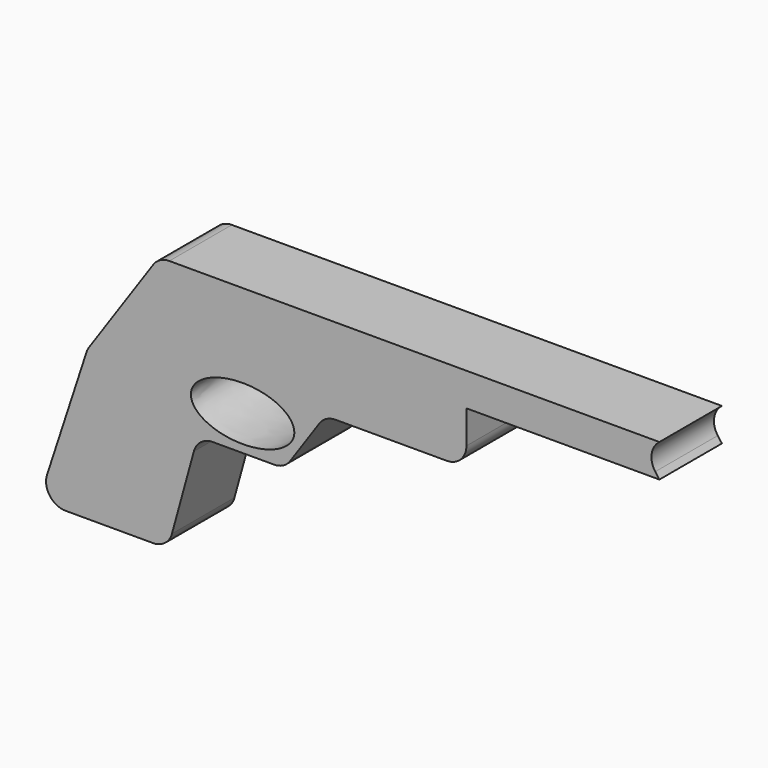
from build123d import *

# Parameters (mm, degrees)
F1_DEPTH = 25.4
F3_DEPTH = 25.4
F4_DEPTH = 25.4


# Not quite as in the source:
# - a feature names something its author has since deleted; it is built from what else it names


with BuildPart() as f1:
    # F0 (on Front) → F1 (new body)
    with BuildSketch(Plane.XZ):
        with BuildLine():
            Line((84.3741819263, 30.5474363267), (21.6592755169, 30.5474363267))
            Line((21.6592755169, 30.5474363267), (21.6592755169, 19.7983730762))
            Line((21.6592755169, 19.7983730762), (84.3741819263, 19.7983730762))
            Line((84.3741819263, 19.7983730762), (83.0258661007, 21.6186676974))
            ThreePointArc((83.0258661007, 21.6186676974), (81.8166137912, 26.0927593628), (83.9697137101, 30.196897289))
            Line((83.9697137101, 30.196897289), (84.3741819263, 30.5474363267))
        make_face()
        with BuildLine():
            Line((21.6592755169, 19.7983730762), (21.6592755169, 30.5474363267))
            Line((21.6592755169, 30.5474363267), (-74.8867837768, 30.5474363267))
            ThreePointArc((-74.8867837768, 30.5474363267), (-77.8464272175, 29.8155330422), (-80.1238115226, 27.7885420603))
            Line((-80.1238115226, 27.7885420603), (-100.9918020349, -2.643935684))
            ThreePointArc((-100.9918020349, -2.643935684), (-101.4491934819, -3.425043187), (-101.7908767788, -4.2632486461))
            Line((-101.7908767788, -4.2632486461), (-114.6295490787, -43.5653208295))
            ThreePointArc((-114.6295490787, -43.5653208295), (-113.7336500917, -49.2654923305), (-108.593446589, -51.887113601))
            Line((-108.593446589, -51.887113601), (-80.1609597975, -51.887113601))
            ThreePointArc((-80.1609597975, -51.887113601), (-76.3124250948, -50.5879828967), (-74.0386146752, -47.2221626222))
            Line((-74.0386146752, -47.2221626222), (-66.9082951101, -21.3153334082))
            ThreePointArc((-66.9082951101, -21.3153334082), (-64.6344846905, -17.9495131337), (-60.7859499878, -16.6503824294))
            Line((-60.7859499878, -16.6503824294), (-40.8448504228, -16.6503824294))
            ThreePointArc((-40.8448504228, -16.6503824294), (-37.8852069821, -15.9184791448), (-35.607822677, -13.8914881629))
            Line((-35.607822677, -13.8914881629), (-26.1230860721, -0.0595844409))
            ThreePointArc((-26.1230860721, -0.0595844409), (-23.845701767, 1.967406541), (-20.8860583263, 2.6993098256))
            Line((-20.8860583263, 2.6993098256), (15.3092755169, 2.6993098256))
            ThreePointArc((15.3092755169, 2.6993098256), (19.7994035774, 4.5591817651), (21.6592755169, 9.0493098256))
            Line((21.6592755169, 9.0493098256), (21.6592755169, 19.7983730762))
        make_face()
    extrude(amount=F1_DEPTH)

    # F2 (on Front) → F3 (join)
    with BuildSketch(Plane.XZ):
        with BuildLine():
            add(Edge.make_bspline(
                [(-61.0972069937, 1.6932484379), (-67.8872726858, -0.9318532182), (-67.8872726858, -5.3358376026)],
                knots=[5.35099187, 5.35099187, 5.35099187, 6.2831853072, 6.2831853072, 6.2831853072], degree=2, weights=[1, 0.8933292345, 1]))
            add(Edge.make_bspline(
                [(-67.8872726858, -5.3358376026), (-67.8872726858, -32.3137216), (-37.4698541145, -10.4760980565), (-7.0524355433, 11.3615254871), (-56.2960408601, 2.9858730785)],
                knots=[0, 0, 0, 2.5140348645, 2.5140348645, 5.028069729, 5.028069729, 5.028069729], degree=2, weights=[1, 0.3086552179, 1, 0.3086552179, 1]))
            Line((-56.2960408601, 2.9858730785), (-51.4948747264, -11.1421316456))
            Line((-51.4948747264, -11.1421316456), (-61.0972069937, 1.6932484379))
        make_face()
        with BuildLine():
            Line((-51.4948747264, -11.1421316456), (-56.2960408601, 2.9858730785))
            add(Edge.make_bspline(
                [(-56.2960408601, 2.9858730785), (-58.8987667134, 2.5431856082), (-61.0972069937, 1.6932484379)],
                knots=[5.028069729, 5.028069729, 5.028069729, 5.35099187, 5.35099187, 5.35099187], degree=2, weights=[1, 0.9869934546, 1]))
            Line((-61.0972069937, 1.6932484379), (-51.4948747264, -11.1421316456))
        make_face()
    extrude(amount=F3_DEPTH)

    # F2 (on Front) → F4 (cut)
    with BuildSketch(Plane.XZ):
        with BuildLine():
            add(Edge.make_bspline(
                [(-61.0972069937, 1.6932484379), (-67.8872726858, -0.9318532182), (-67.8872726858, -5.3358376026)],
                knots=[5.35099187, 5.35099187, 5.35099187, 6.2831853072, 6.2831853072, 6.2831853072], degree=2, weights=[1, 0.8933292345, 1]))
            add(Edge.make_bspline(
                [(-67.8872726858, -5.3358376026), (-67.8872726858, -32.3137216), (-37.4698541145, -10.4760980565), (-7.0524355433, 11.3615254871), (-56.2960408601, 2.9858730785)],
                knots=[0, 0, 0, 2.5140348645, 2.5140348645, 5.028069729, 5.028069729, 5.028069729], degree=2, weights=[1, 0.3086552179, 1, 0.3086552179, 1]))
            Line((-56.2960408601, 2.9858730785), (-51.4948747264, -11.1421316456))
            Line((-51.4948747264, -11.1421316456), (-61.0972069937, 1.6932484379))
        make_face()
        with BuildLine():
            Line((-51.4948747264, -11.1421316456), (-56.2960408601, 2.9858730785))
            add(Edge.make_bspline(
                [(-56.2960408601, 2.9858730785), (-58.8987667134, 2.5431856082), (-61.0972069937, 1.6932484379)],
                knots=[5.028069729, 5.028069729, 5.028069729, 5.35099187, 5.35099187, 5.35099187], degree=2, weights=[1, 0.9869934546, 1]))
            Line((-61.0972069937, 1.6932484379), (-51.4948747264, -11.1421316456))
        make_face()
    extrude(amount=F4_DEPTH, mode=Mode.SUBTRACT)


solid = f1.part
